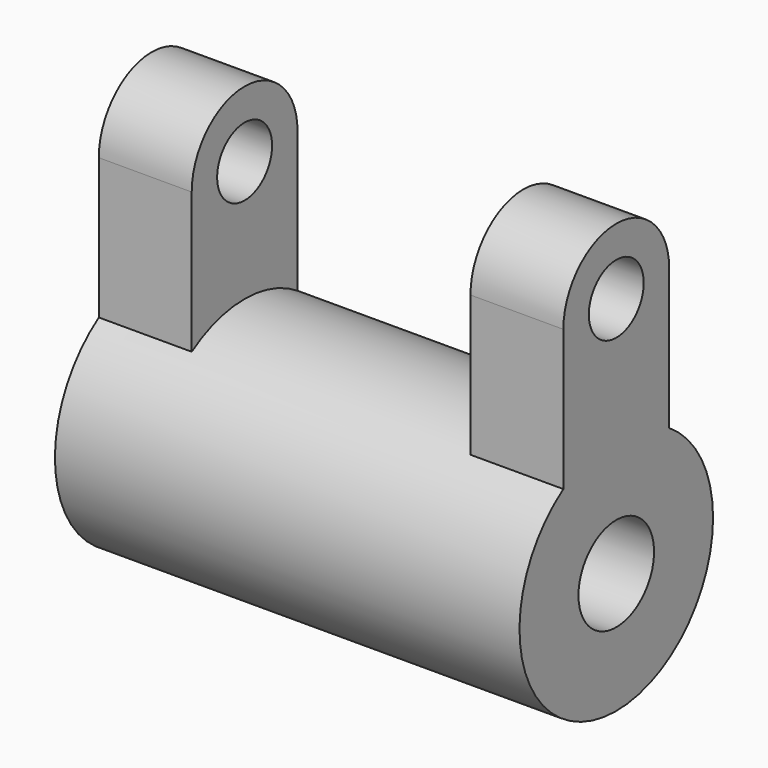
from build123d import *

# Parameters (mm, degrees)
F0_R      = 33.0702193876
F1_DEPTH  = 63.5
F3_DEPTH  = 25.4
F7_DEPTH  = 25.4
F8_DEPTH  = 25.4
F9_R      = 12.915127355
F10_DEPTH = 127.001
F11_R     = 9.381167956
F12_DEPTH = 127.001


with BuildPart() as f1:
    # F0 (on Right) → F1 (new body)
    with BuildSketch(Plane.YZ):
        Circle(F0_R)
    extrude(amount=-F1_DEPTH)

    # F2 (on face) → F3 (join)
    with BuildSketch(Plane.YZ):
        with BuildLine():
            Line((-18.0798303336, 66.1404387753), (-18.0798303336, 27.69041613))
            ThreePointArc((-18.0798303336, 27.69041613), (0, 33.0702193876), (18.0798303336, 27.69041613))
            Line((18.0798303336, 27.69041613), (18.0798303336, 66.1404387753))
            Line((18.0798303336, 66.1404387753), (-18.0798303336, 66.1404387753))
        make_face()
        with BuildLine():
            Line((-18.0798303336, 27.69041613), (-18.0798303336, 0))
            Line((-18.0798303336, 0), (18.0798303336, 0))
            Line((18.0798303336, 0), (18.0798303336, 27.69041613))
            ThreePointArc((18.0798303336, 27.69041613), (0, 33.0702193876), (-18.0798303336, 27.69041613))
        make_face()
    extrude(amount=-F3_DEPTH)

    # F4: F1 across face


with BuildPart() as f1_1:
    add(f1.part)
    add(f1.part.mirror(Plane(origin=(-63.5, 0, 0), x_dir=(0, 1, 0), z_dir=(-1, 0, 0))))

    # F5 (on face) → F7 (join)
    with BuildSketch(Plane.YZ):
        with BuildLine():
            ThreePointArc((-18.0798303336, 66.1404387753), (0, 48.0606084417), (18.0798303336, 66.1404387753))
            Line((18.0798303336, 66.1404387753), (-18.0798303336, 66.1404387753))
        make_face()
        with BuildLine():
            Line((-18.0798303336, 66.1404387753), (18.0798303336, 66.1404387753))
            ThreePointArc((18.0798303336, 66.1404387753), (0, 84.2202691088), (-18.0798303336, 66.1404387753))
        make_face()
    extrude(amount=-F7_DEPTH)

    # F6 (on face) → F8 (join)
    with BuildSketch(Plane(origin=(-127, 0, 0), x_dir=(0, -1, 0), z_dir=(-1, 0, 0))):
        with BuildLine():
            Line((-18.0798303336, 66.1404387753), (18.0798303336, 66.1404387753))
            ThreePointArc((18.0798303336, 66.1404387753), (0, 84.2202691088), (-18.0798303336, 66.1404387753))
        make_face()
    extrude(amount=-F8_DEPTH)

    # F9 (on face) → F10 (cut, through all)
    with BuildSketch(Plane(origin=(-127, 0, 0), x_dir=(0, -1, 0), z_dir=(-1, 0, 0))):
        Circle(F9_R)
    extrude(amount=-F10_DEPTH, mode=Mode.SUBTRACT)

    # F11 (on face) → F12 (cut, through all)
    with BuildSketch(Plane.YZ):
        with Locations((0, 66.1404387753)):
            Circle(F11_R)
    extrude(amount=-F12_DEPTH, mode=Mode.SUBTRACT)


solid = f1_1.part
